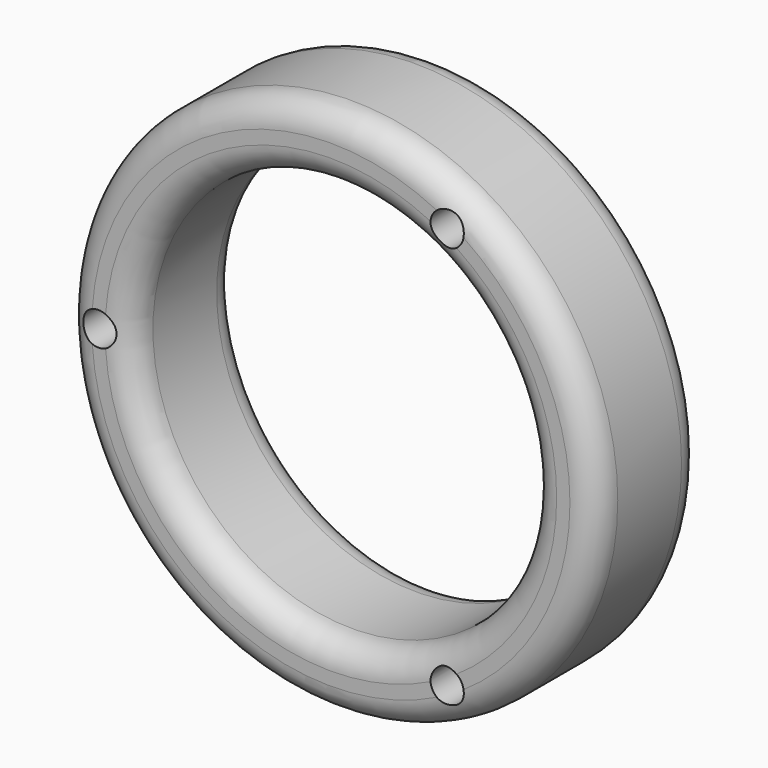
from build123d import *

# Parameters (mm, degrees)
F0_R     = 50.8
F0_R_2   = 3.175
F0_R_3   = 38.1
F1_DEPTH = 25.4


# Not quite as in the source:
# - a fillet or chamfer that OpenCascade refuses, or shapes differently, is made with other operations: its cross-section is extruded or revolved along the edge and cut away or added


with BuildPart() as f1:
    # F0 (on Front) → F1 (new body)
    with BuildSketch(Plane.XZ):
        Circle(F0_R)
        with Locations((-44.45, 0)):
            Circle(F0_R_2, mode=Mode.SUBTRACT)
        Circle(F0_R_3, mode=Mode.SUBTRACT)
        with Locations((22.225, -38.4948291982)):
            Circle(F0_R_2, mode=Mode.SUBTRACT)
        with Locations((22.225, 38.4948291982)):
            Circle(F0_R_2, mode=Mode.SUBTRACT)
    extrude(amount=F1_DEPTH)

    # F2: fillet of radius 5.08 on 4 edges, made by hand

    # F2_s1 → F2_t2 (revolve, cut)
    with BuildSketch(Plane.XY):
        with BuildLine():
            ThreePointArc((50.8, -5.08), (49.3121024484, -1.4878975516), (45.72, 0))
            Line((45.72, 0), (50.8, 0))
            Line((50.8, 0), (50.8, -5.08))
        make_face()
    revolve(axis=Axis((0, 0, 0), (0, -1, 0)), mode=Mode.SUBTRACT)

    # F2_s3 → F2_t4 (revolve, cut)
    with BuildSketch(Plane.XY):
        with BuildLine():
            ThreePointArc((38.1, -5.08), (39.5878975516, -1.4878975516), (43.18, 0))
            Line((43.18, 0), (38.1, 0))
            Line((38.1, 0), (38.1, -5.08))
        make_face()
    revolve(axis=Axis((0, 0, 0), (0, -1, 0)), mode=Mode.SUBTRACT)

    # F2_s5 → F2_t6 (revolve, cut)
    with BuildSketch(Plane.XY):
        with BuildLine():
            ThreePointArc((38.1, -20.32), (39.5878975516, -23.9121024484), (43.18, -25.4))
            Line((43.18, -25.4), (38.1, -25.4))
            Line((38.1, -25.4), (38.1, -20.32))
        make_face()
    revolve(axis=Axis((0, -25.4, 0), (0, -1, 0)), mode=Mode.SUBTRACT)

    # F2_s7 → F2_t8 (revolve, cut)
    with BuildSketch(Plane.XY):
        with BuildLine():
            ThreePointArc((50.8, -20.32), (49.3121024484, -23.9121024484), (45.72, -25.4))
            Line((45.72, -25.4), (50.8, -25.4))
            Line((50.8, -25.4), (50.8, -20.32))
        make_face()
    revolve(axis=Axis((0, -25.4, 0), (0, -1, 0)), mode=Mode.SUBTRACT)


solid = f1.part
